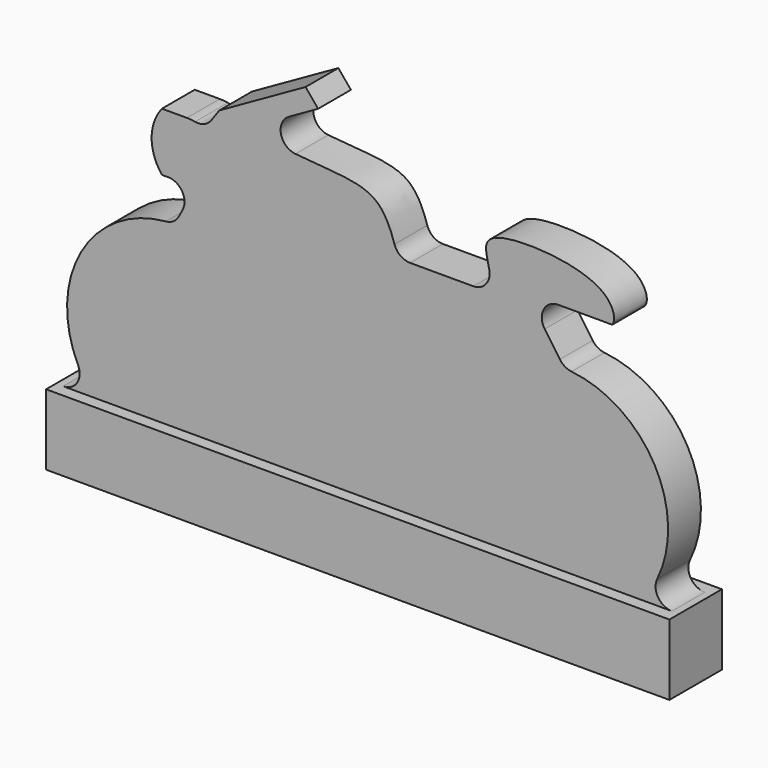
from build123d import *

# Parameters (mm, degrees)
F0_W          = 152
F0_H          = 118
F1_DEPTH      = 10
F3_DEPTH      = 10.001
F5_W          = 152
F5_H          = 17.2627116575
F6_DEPTH      = 8
F6_DEPTH_BACK = 8


# Not quite as in the source:
# - a feature of the source that left no trace in its solid (it failed there, or was rolled back) is left out


with BuildPart() as f1:
    # F0 (on Front) → F1 (new body)
    with BuildSketch(Plane.XZ):
        Rectangle(F0_W, F0_H)
    extrude(amount=F1_DEPTH)

    # F2 (on face) → F3 (cut, through all)
    with BuildSketch(Plane.XZ.offset(10)):
        with BuildLine():
            ThreePointArc((-70.6181125347, -35.9849638434), (-69.8524168033, -11.4609840482), (-49.1986901165, 1.7842207028))
            ThreePointArc((-49.1986901165, 1.7842207028), (-47.3292301622, 2.4363845666), (-46.0015605766, 3.9052248226))
            Line((-46.0015605766, 3.9052248226), (-45.1064301329, 5.6043666467))
            ThreePointArc((-45.1064301329, 5.6043666467), (-45.2206540403, 9.5354363514), (-48.6453771591, 11.4687308669))
            Line((-48.6453771591, 11.4687308669), (-50.1535981894, 11.4687308669))
            ThreePointArc((-50.1535981894, 11.4687308669), (-52.6629001179, 18.5783598579), (-50.1535981894, 25.6879888489))
            Line((-50.1535981894, 25.6879888489), (-44.0518481356, 25.6879888489))
            ThreePointArc((-44.0518481356, 25.6879888489), (-43.059526136, 25.6424430426), (-42.0755484424, 25.5061886123))
            ThreePointArc((-42.0755484424, 25.5061886123), (-39.8317724868, 25.736665969), (-38.0694248209, 27.1444234254))
            Line((-38.0694248209, 27.1444234254), (-36.1724459248, 29.8530095604))
            Line((-36.1724459248, 29.8530095604), (-15.1238283804, 41.7308993996))
            Line((-15.1238283804, 41.7308993996), (-12.0670144845, 38.0450352231))
            Line((-12.0670144845, 38.0450352231), (-19.1861068518, 34.0276789898))
            ThreePointArc((-19.1861068518, 34.0276789898), (-21.1323066606, 29.7097716233), (-17.5938420386, 26.5615521519))
            add(Edge.make_bspline(
                [(6.5517873057, 15.0364702316), (5.491363759, 18.3398524068), (2.2668782528, 25.5558310957), (-7.9913531629, 25.6427173347), (-16.3640968599, 26.4462017738), (-17.5938420386, 26.5615521519)],
                knots=[0.0475862763, 0.0475862763, 0.0475862763, 0.0475862763, 0.2218165071, 0.4786686805, 0.5223610745, 0.5223610745, 0.5223610745, 0.5223610745], degree=3))
            ThreePointArc((6.5517873057, 15.0364702316), (8.0035004043, 13.027164561), (10.360364081, 12.2590670362))
            Line((10.360364081, 12.2590670362), (25.7659908384, 12.2590670362))
            ThreePointArc((25.7659908384, 12.2590670362), (28.9109617934, 13.7873960038), (29.652657642, 17.2044881901))
            add(Edge.make_bspline(
                [(59.659762206, 15.0137214134), (60.6116106124, 16.3891165896), (58.9310149138, 23.1502612618), (41.0901009905, 26.3300404656), (29.1222511268, 24.7385599898), (28.6760066521, 21.1229006979), (29.3934875571, 18.2699474948), (29.652657642, 17.2044881901)],
                knots=[0, 0, 0, 0, 0.1654357838, 0.4540176091, 0.6794036074, 0.807442682, 0.8805736461, 0.8805736461, 0.8805736461, 0.8805736461], degree=3))
            Line((59.659762206, 15.0137214134), (46.4762444892, 15.0137214134))
            ThreePointArc((46.4762444892, 15.0137214134), (42.9307573339, 12.8656179633), (43.1933067739, 8.7284818292))
            Line((43.1933067739, 8.7284818292), (46.8858224383, 3.4238743724))
            ThreePointArc((46.8858224383, 3.4238743724), (48.1310071639, 2.267085085), (49.7440886364, 1.731721079))
            ThreePointArc((49.7440886364, 1.731721079), (69.9863232581, -11.6999924827), (70.6181125348, -35.9849638434))
            ThreePointArc((70.6181125348, -35.9849638434), (70.8220039214, -39.8575126235), (74.2138543011, -41.7372883425))
            Line((74.2138543011, -41.7372883425), (76, -41.7372883425))
            Line((76, -41.7372883425), (76, 59))
            Line((76, 59), (-76, 59))
            Line((-76, 59), (-76, -41.7372883425))
            Line((-76, -41.7372883425), (-74.213854301, -41.7372883425))
            ThreePointArc((-74.213854301, -41.7372883425), (-70.8220039214, -39.8575126235), (-70.6181125347, -35.9849638434))
        make_face()
    extrude(amount=-F3_DEPTH, mode=Mode.SUBTRACT)

    # F5 (on mid) → F6 (join, two sides)
    with BuildSketch(Plane.XZ.offset(5)) as f6_sk:
        with Locations((0, -50.3686441713)):
            Rectangle(F5_W, F5_H)
    extrude(amount=F6_DEPTH)
    extrude(f6_sk.sketch, amount=-F6_DEPTH_BACK)


solid = f1.part
